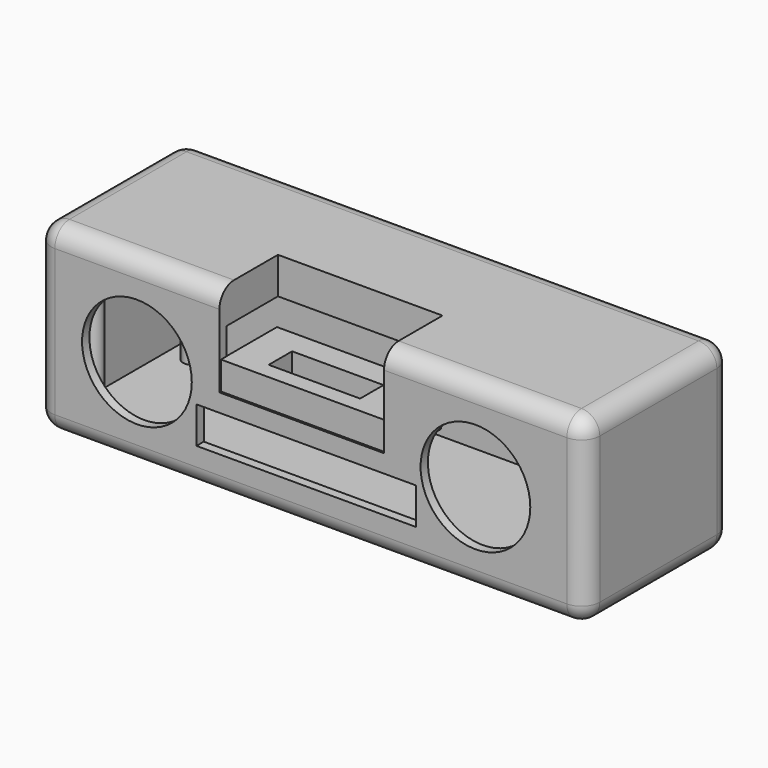
from build123d import *

# Parameters (mm, degrees)
F0_W          = 150
F0_H          = 40
F1_DEPTH      = 50
F2_T          = -2.5
F5_R          = 2.5
F7_DEPTH      = 40
F6_R          = 2.5
F8_DEPTH      = 40
F4_R          = 2.5
F9_DEPTH      = 40
F3_R          = 2.5
F10_DEPTH     = 40
F11_W         = 150
F11_H         = 50
F12_DEPTH     = 10
F13_W         = 45
F13_H         = 20
F14_DEPTH     = 25
F15_W         = 44.8060352355
F15_H         = 19.2025862634
F16_DEPTH     = 10
F17_W         = 25
F17_H         = 8
F18_DEPTH     = 25
F19_R         = 15
F20_DEPTH     = 5
F21_R         = 5
F22_T1_DEPTH  = 57.5
F22_T3_DEPTH  = 40
F22_T5_DEPTH  = 57.5
F22_T7_DEPTH  = 40
F22_S11_W     = 5
F22_S11_H     = 5
F22_T12_DEPTH = 5
F22_S17_W     = 5
F22_S17_H     = 5
F22_T18_DEPTH = 5
F22_S23_W     = 5
F22_S23_H     = 5
F22_T24_DEPTH = 5
F22_S29_W     = 5
F22_S29_H     = 5
F22_T30_DEPTH = 5
F22_T34_ANGLE = 90
F22_T36_ANGLE = 90
F22_T38_ANGLE = 90
F23_T1_DEPTH  = 62.5
F23_S5_W      = 5
F23_S5_H      = 5
F23_T6_DEPTH  = 5
F24_W         = 60
F24_H         = 10
F25_DEPTH     = 25


# Not quite as in the source:
# - a fillet or chamfer that OpenCascade refuses, or shapes differently, is made with other operations: its cross-section is extruded or revolved along the edge and cut away or added


with BuildPart() as f1:
    # F0 (on Front) → F1 (new body)
    with BuildSketch(Plane.XZ):
        with Locations((-1.4870658517, -2.6939674467)):
            Rectangle(F0_W, F0_H)
    extrude(amount=F1_DEPTH)

    # F2
    f2_openings = [f1.faces().sort_by_distance(p)[0] for p in [
        (-1.487066, -25, 17.306033),
    ]]
    offset(amount=F2_T, openings=f2_openings)

    # F5 (on face) → F7 (join)
    with BuildSketch(Plane.XY.offset(-20.1939674467)):
        with Locations((64.5129341483, -42)):
            Circle(F5_R)
    extrude(amount=F7_DEPTH)

    # F6 (on face) → F8 (join)
    with BuildSketch(Plane.XY.offset(-20.1939674467)):
        with Locations((-67.4870658517, -42)):
            Circle(F6_R)
    extrude(amount=F8_DEPTH)

    # F4 (on face) → F9 (join)
    with BuildSketch(Plane.XY.offset(-20.1939674467)):
        with Locations((64.5129341483, -8)):
            Circle(F4_R)
    extrude(amount=F9_DEPTH)

    # F3 (on face) → F10 (join)
    with BuildSketch(Plane.XY.offset(-20.1939674467)):
        with Locations((-67.4870658517, -8)):
            Circle(F3_R)
    extrude(amount=F10_DEPTH)

    # F11 (on face) → F12 (join)
    with BuildSketch(Plane.XY.offset(17.3060325533)):
        with Locations((-1.4870658517, -25)):
            Rectangle(F11_W, F11_H)
    extrude(amount=F12_DEPTH)

    # F13 (on face) → F14 (cut)
    with BuildSketch(Plane.XY.offset(27.3060325533)):
        with Locations((-3.9870658517, -40)):
            Rectangle(F13_W, F13_H)
    extrude(amount=-F14_DEPTH, mode=Mode.SUBTRACT)

    # F15 (on Top) → F16 (join)
    with BuildSketch(Plane.XY):
        with Locations((-4.1379285976, -39.8599151522)):
            Rectangle(F15_W, F15_H)
    extrude(amount=F16_DEPTH)

    # F17 (on face) → F18 (cut)
    with BuildSketch(Plane.XY.offset(10)):
        with Locations((-4.5150823891, -41.0000055134)):
            Rectangle(F17_W, F17_H)
    extrude(amount=-F18_DEPTH, mode=Mode.SUBTRACT)

    # F19 (on face) → F20 (cut)
    with BuildSketch(Plane.XZ.offset(50)):
        with Locations((-49.0409471095, 2.3060325533)):
            Circle(F19_R)
        with Locations((43.5129341483, 2.3060325533)):
            Circle(F19_R)
    extrude(amount=-F20_DEPTH, mode=Mode.SUBTRACT)

    # F21
    f21_edges = [f1.edges().sort_by_distance(p)[0] for p in [
        (-1.487066, -50, -22.693967),
        (73.512934, -25, -22.693967),
        (-76.487066, -25, -22.693967),
        (-1.487066, 0, -22.693967),
        (-1.487066, 0, 27.306033),
        (-51.487066, -50, 27.306033),
    ]]
    fillet(f21_edges, radius=F21_R)

    # F22: fillet of radius 5 on 3 edges, made by hand

    # F22_s2 → F22_t1 (cut)
    with BuildSketch(Plane.XZ.offset(5)):
        with BuildLine():
            ThreePointArc((68.5129341483, 27.3060325533), (72.0484680542, 25.8415664592), (73.5129341483, 22.3060325533))
            Line((73.5129341483, 22.3060325533), (73.5129341483, 27.3060325533))
            Line((73.5129341483, 27.3060325533), (68.5129341483, 27.3060325533))
        make_face()
    extrude(amount=F22_T1_DEPTH, mode=Mode.SUBTRACT)

    # F22_s4 → F22_t3 (cut)
    with BuildSketch(Plane.XZ.offset(5)):
        with BuildLine():
            ThreePointArc((-76.4870658517, 22.3060325533), (-75.0225997576, 25.8415664592), (-71.4870658517, 27.3060325533))
            Line((-71.4870658517, 27.3060325533), (-76.4870658517, 27.3060325533))
            Line((-76.4870658517, 27.3060325533), (-76.4870658517, 22.3060325533))
        make_face()
    extrude(amount=F22_T3_DEPTH, mode=Mode.SUBTRACT)

    # F22_s6 → F22_t5 (cut)
    with BuildSketch(Plane.XY.offset(-17.6939674467)):
        with BuildLine():
            ThreePointArc((68.5129341483, -50), (72.0484680542, -48.5355339059), (73.5129341483, -45))
            Line((73.5129341483, -45), (73.5129341483, -50))
            Line((73.5129341483, -50), (68.5129341483, -50))
        make_face()
    extrude(amount=F22_T5_DEPTH, mode=Mode.SUBTRACT)

    # F22_s8 → F22_t7 (cut)
    with BuildSketch(Plane.XY.offset(-17.6939674467)):
        with BuildLine():
            ThreePointArc((-76.4870658517, -45), (-75.0225997576, -48.5355339059), (-71.4870658517, -50))
            Line((-71.4870658517, -50), (-76.4870658517, -50))
            Line((-76.4870658517, -50), (-76.4870658517, -45))
        make_face()
        with BuildLine():
            ThreePointArc((-76.4870658517, -5), (-75.0225997576, -1.4644660941), (-71.4870658517, 0))
            Line((-71.4870658517, 0), (-76.4870658517, 0))
            Line((-76.4870658517, 0), (-76.4870658517, -5))
        make_face()
        with BuildLine():
            ThreePointArc((68.5129341483, 0), (72.0484680542, -1.4644660941), (73.5129341483, -5))
            Line((73.5129341483, -5), (73.5129341483, 0))
            Line((73.5129341483, 0), (68.5129341483, 0))
        make_face()
    extrude(amount=F22_T7_DEPTH, mode=Mode.SUBTRACT)


with BuildPart() as f22_tool10:
    # F22_s11 → F22_t12 (new body)
    with BuildSketch(Plane.XZ.offset(45)):
        with Locations((71.0129341483, -20.1939674467)):
            Rectangle(F22_S11_W, F22_S11_H)
    extrude(amount=F22_T12_DEPTH)

    # F22_s13 → F22_t14 (revolve, cut)
    with BuildSketch(Plane(origin=(68.5129341483, -45, -17.6939674467), x_dir=(-0.7071067812, 0, 0.7071067812), z_dir=(0.7071067812, 0, 0.7071067812))):
        with BuildLine():
            ThreePointArc((0, -5), (5, 0), (0, 5))
            Line((0, 5), (0, -5))
        make_face()
    revolve(axis=Axis((68.5129341483, -45, -17.6939674467), (0, -1, 0)), mode=Mode.SUBTRACT)


with BuildPart() as f1_1:
    add(f1.part)

    # F22_t9: cut F22_tool10
    add(f22_tool10.part, mode=Mode.SUBTRACT)


with BuildPart() as f22_tool16:
    # F22_s17 → F22_t18 (new body)
    with BuildSketch(Plane.YZ.offset(-71.4870658517)):
        with Locations((-47.5, -20.1939674467)):
            Rectangle(F22_S17_W, F22_S17_H)
    extrude(amount=-F22_T18_DEPTH)

    # F22_s19 → F22_t20 (revolve, cut)
    with BuildSketch(Plane(origin=(-71.4870658517, -45, -17.6939674467), x_dir=(0, 0.7071067812, 0.7071067812), z_dir=(0, -0.7071067812, 0.7071067812))):
        with BuildLine():
            ThreePointArc((0, -5), (5, 0), (0, 5))
            Line((0, 5), (0, -5))
        make_face()
    revolve(axis=Axis((-71.4870658517, -45, -17.6939674467), (-1, 0, 0)), mode=Mode.SUBTRACT)


with BuildPart() as f1_2:
    add(f1_1.part)

    # F22_t15: cut F22_tool16
    add(f22_tool16.part, mode=Mode.SUBTRACT)


with BuildPart() as f22_tool22:
    # F22_s23 → F22_t24 (new body)
    with BuildSketch(Plane.YZ.offset(-71.4870658517)):
        with Locations((-2.5, -20.1939674467)):
            Rectangle(F22_S23_W, F22_S23_H)
    extrude(amount=-F22_T24_DEPTH)

    # F22_s25 → F22_t26 (revolve, cut)
    with BuildSketch(Plane(origin=(-71.4870658517, -5, -17.6939674467), x_dir=(0, -0.7071067812, 0.7071067812), z_dir=(0, -0.7071067812, -0.7071067812))):
        with BuildLine():
            ThreePointArc((0, -5), (5, 0), (0, 5))
            Line((0, 5), (0, -5))
        make_face()
    revolve(axis=Axis((-71.4870658517, -5, -17.6939674467), (-1, 0, 0)), mode=Mode.SUBTRACT)


with BuildPart() as f1_3:
    add(f1_2.part)

    # F22_t21: cut F22_tool22
    add(f22_tool22.part, mode=Mode.SUBTRACT)


with BuildPart() as f22_tool28:
    # F22_s29 → F22_t30 (new body)
    with BuildSketch(Plane.XZ.offset(5)):
        with Locations((71.0129341483, -20.1939674467)):
            Rectangle(F22_S29_W, F22_S29_H)
    extrude(amount=-F22_T30_DEPTH)

    # F22_s31 → F22_t32 (revolve, cut)
    with BuildSketch(Plane(origin=(68.5129341483, -5, -17.6939674467), x_dir=(-0.7071067812, 0, 0.7071067812), z_dir=(-0.7071067812, 0, -0.7071067812))):
        with BuildLine():
            ThreePointArc((0, -5), (5, 0), (0, 5))
            Line((0, 5), (0, -5))
        make_face()
    revolve(axis=Axis((68.5129341483, -5, -17.6939674467), (0, 1, 0)), mode=Mode.SUBTRACT)


with BuildPart() as f1_4:
    add(f1_3.part)

    # F22_t27: cut F22_tool28
    add(f22_tool28.part, mode=Mode.SUBTRACT)

    # F22_s33 → F22_t34 (revolve, cut)
    with BuildSketch(Plane.XY.offset(22.3060325533)):
        with BuildLine():
            ThreePointArc((-76.4870658517, -5), (-75.0225997576, -1.4644660941), (-71.4870658517, 0))
            Line((-71.4870658517, 0), (-76.4870658517, 0))
            Line((-76.4870658517, 0), (-76.4870658517, -5))
        make_face()
    revolve(axis=Axis((-76.4870658517, -5, 22.3060325533), (1, 0, 0)), revolution_arc=F22_T34_ANGLE, mode=Mode.SUBTRACT)

    # F22_s35 → F22_t36 (revolve, cut)
    with BuildSketch(Plane.XZ.offset(45)):
        with BuildLine():
            ThreePointArc((-76.4870658517, 22.3060325533), (-75.0225997576, 25.8415664592), (-71.4870658517, 27.3060325533))
            Line((-71.4870658517, 27.3060325533), (-76.4870658517, 27.3060325533))
            Line((-76.4870658517, 27.3060325533), (-76.4870658517, 22.3060325533))
        make_face()
    revolve(axis=Axis((-76.4870658517, -45, 22.3060325533), (1, 0, 0)), revolution_arc=F22_T36_ANGLE, mode=Mode.SUBTRACT)

    # F22_s37 → F22_t38 (revolve, cut)
    with BuildSketch(Plane.XY.offset(22.3060325533)):
        with BuildLine():
            ThreePointArc((68.5129341483, 0), (72.0484680542, -1.4644660941), (73.5129341483, -5))
            Line((73.5129341483, -5), (73.5129341483, 0))
            Line((73.5129341483, 0), (68.5129341483, 0))
        make_face()
    revolve(axis=Axis((73.5129341483, -5, 22.3060325533), (1, 0, 0)), revolution_arc=F22_T38_ANGLE, mode=Mode.SUBTRACT)

    # F23: fillet of radius 5 on 1 edges, made by hand

    # F23_s2 → F23_t1 (cut)
    with BuildSketch(Plane.YZ.offset(6.0129341483)):
        with BuildLine():
            ThreePointArc((-50, 22.3060325533), (-48.5355339059, 25.8415664592), (-45, 27.3060325533))
            Line((-45, 27.3060325533), (-50, 27.3060325533))
            Line((-50, 27.3060325533), (-50, 22.3060325533))
        make_face()
    extrude(amount=F23_T1_DEPTH, mode=Mode.SUBTRACT)


with BuildPart() as f23_tool4:
    # F23_s5 → F23_t6 (new body)
    with BuildSketch(Plane.XZ.offset(45)):
        with Locations((71.0129341483, 24.8060325533)):
            Rectangle(F23_S5_W, F23_S5_H)
    extrude(amount=F23_T6_DEPTH)

    # F23_s7 → F23_t8 (revolve, cut)
    with BuildSketch(Plane(origin=(68.5129341483, -45, 22.3060325533), x_dir=(-0.7071067812, 0, -0.7071067812), z_dir=(-0.7071067812, 0, 0.7071067812))):
        with BuildLine():
            ThreePointArc((0, -5), (5, 0), (0, 5))
            Line((0, 5), (0, -5))
        make_face()
    revolve(axis=Axis((68.5129341483, -45, 22.3060325533), (0, -1, 0)), mode=Mode.SUBTRACT)


with BuildPart() as f1_5:
    add(f1_4.part)

    # F23_t3: cut F23_tool4
    add(f23_tool4.part, mode=Mode.SUBTRACT)

    # F24 (on face) → F25 (cut)
    with BuildSketch(Plane.XZ.offset(50)):
        with Locations((-2.7640064806, -7.5991895379)):
            Rectangle(F24_W, F24_H)
    extrude(amount=-F25_DEPTH, mode=Mode.SUBTRACT)


solid = f1_5.part
